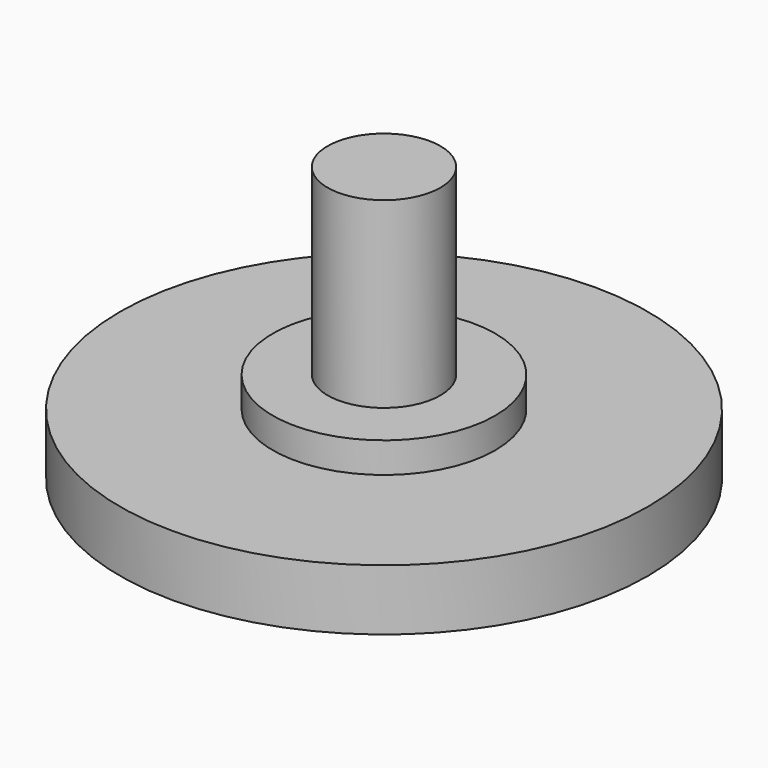
from build123d import *

# Parameters (mm, degrees)
F0_R        = 2.35
F1_DEPTH    = 11.43
F0_R_2      = 4.636
F2_DEPTH    = 3.81
F0_R_3      = 11
F3_DEPTH    = 2.54
F5_DEPTH    = 1.27
F6_T1_DEPTH = 12.7
F6_T3_DEPTH = 7.62
F6_T5_DEPTH = 4.445
F6_T7_DEPTH = 4.079017898
F6_T9_DEPTH = 6.0188206533


# Not quite as in the source:
# - a fillet or chamfer that OpenCascade refuses, or shapes differently, is made with other operations: its cross-section is extruded or revolved along the edge and cut away or added


with BuildPart() as f1:
    # F0 (on Top) → F1 (new body)
    with BuildSketch(Plane.XY):
        Circle(F0_R)
    extrude(amount=F1_DEPTH)

    # F0 (on Top) → F2 (join)
    with BuildSketch(Plane.XY):
        Circle(F0_R_2)
        Circle(F0_R, mode=Mode.SUBTRACT)
    extrude(amount=F2_DEPTH)

    # F0 (on Top) → F3 (join)
    with BuildSketch(Plane.XY):
        Circle(F0_R_3)
        Circle(F0_R_2, mode=Mode.SUBTRACT)
    extrude(amount=F3_DEPTH)

    # F4 (on face) → F5 (join)
    with BuildSketch(Plane.XY):
        with BuildLine():
            ThreePointArc((0, -6.7733326328), (-6.1696334492, -0.6777773574), (0, 5.417777918))
            ThreePointArc((0, 5.417777918), (1.9417265012, 4.2834880284), (2.4694073737, 2.0975172472))
            Line((2.4694073737, 2.0975172472), (4.8922184175, 2.0975172472))
            ThreePointArc((4.8922184175, 2.0975172472), (3.5875761059, 5.9808584475), (0, 7.9586673672))
            ThreePointArc((0, 7.9586673672), (-8.382, -0.4233326328), (0, -8.8053326328))
            ThreePointArc((0, -8.8053326328), (3.39954986, -7.3527295439), (5.0117596984, -4.0259030648))
            Line((5.0117596984, -4.0259030648), (2.4717596984, -4.0259030648))
            ThreePointArc((2.4717596984, -4.0259030648), (1.8244333866, -5.9291174694), (0, -6.7733326328))
        make_face()
        with BuildLine():
            Line((4.8922184175, 2.0975172472), (2.4694073737, 2.0975172472))
            ThreePointArc((2.4694073737, 2.0975172472), (2.3960471942, 1.7747190007), (2.2859995271, 1.4625172472))
            Line((2.2859995271, 1.4625172472), (4.8259995271, 1.4625172472))
            ThreePointArc((4.8259995271, 1.4625172472), (4.8680955625, 1.7790801102), (4.8922184175, 2.0975172472))
        make_face()
        with BuildLine():
            ThreePointArc((2.2859995271, 1.4625172472), (2.3960471942, 1.7747190007), (2.4694073737, 2.0975172472))
            Line((2.4694073737, 2.0975172472), (0.3809995271, 2.0975172472))
            Line((0.3809995271, 2.0975172472), (0.3809995271, 0.8275172472))
            Line((0.3809995271, 0.8275172472), (6.7309995271, 0.8275172472))
            Line((6.7309995271, 0.8275172472), (6.7309995271, 2.0975172472))
            Line((6.7309995271, 2.0975172472), (4.8922184175, 2.0975172472))
            ThreePointArc((4.8922184175, 2.0975172472), (4.8680955625, 1.7790801102), (4.8259995271, 1.4625172472))
            Line((4.8259995271, 1.4625172472), (2.2859995271, 1.4625172472))
        make_face()
    extrude(amount=-F5_DEPTH)

    # F6: fillet of radius 1.27 on 5 edges, made by hand

    # F6_s2 → F6_t1 (cut)
    with BuildSketch(Plane.YZ.offset(-2.7940004729)):
        with BuildLine():
            ThreePointArc((0.8275172472, 0), (1.1994916351, -0.8980256121), (2.0975172472, -1.27))
            Line((2.0975172472, -1.27), (0.8275172472, -1.27))
            Line((0.8275172472, -1.27), (0.8275172472, 0))
        make_face()
    extrude(amount=F6_T1_DEPTH, mode=Mode.SUBTRACT)

    # F6_s4 → F6_t3 (cut)
    with BuildSketch(Plane.XZ.offset(-5.2725172472)):
        with BuildLine():
            ThreePointArc((6.7309995271, 0), (6.3590251392, -0.8980256121), (5.4609995271, -1.27))
            Line((5.4609995271, -1.27), (6.7309995271, -1.27))
            Line((6.7309995271, -1.27), (6.7309995271, 0))
        make_face()
    extrude(amount=F6_T3_DEPTH, mode=Mode.SUBTRACT)

    # F6_s6 → F6_t5 (cut)
    with BuildSketch(Plane.XZ.offset(-2.0975172472)):
        with BuildLine():
            ThreePointArc((0.3809995271, 0), (0.752973915, -0.8980256121), (1.6509995271, -1.27))
            Line((1.6509995271, -1.27), (0.3809995271, -1.27))
            Line((0.3809995271, -1.27), (0.3809995271, 0))
        make_face()
    extrude(amount=F6_T5_DEPTH, mode=Mode.SUBTRACT)

    # F6_s8 → F6_t7 (cut)
    with BuildSketch(Plane.XY.offset(-4.079017898)):
        with BuildLine():
            ThreePointArc((3.5953668576, -4.0259030648), (2.8338642738, -4.2795301928), (2.3765155692, -4.9391096556))
            ThreePointArc((2.3765155692, -4.9391096556), (2.4655394537, -4.4868244195), (2.4717596984, -4.0259030648))
            Line((2.4717596984, -4.0259030648), (3.5953668576, -4.0259030648))
        make_face()
    extrude(amount=F6_T7_DEPTH, mode=Mode.SUBTRACT)

    # F6_s10 → F6_t9 (cut)
    with BuildSketch(Plane.XY.offset(-6.0188206533)):
        with BuildLine():
            ThreePointArc((4.4971207542, -5.8543872382), (4.4340465678, -4.6237330343), (3.3565088886, -4.0259030648))
            Line((3.3565088886, -4.0259030648), (5.0117596984, -4.0259030648))
            ThreePointArc((5.0117596984, -4.0259030648), (4.837388646, -4.9634915319), (4.4971207542, -5.8543872382))
        make_face()
    extrude(amount=F6_T9_DEPTH, mode=Mode.SUBTRACT)


solid = f1.part
